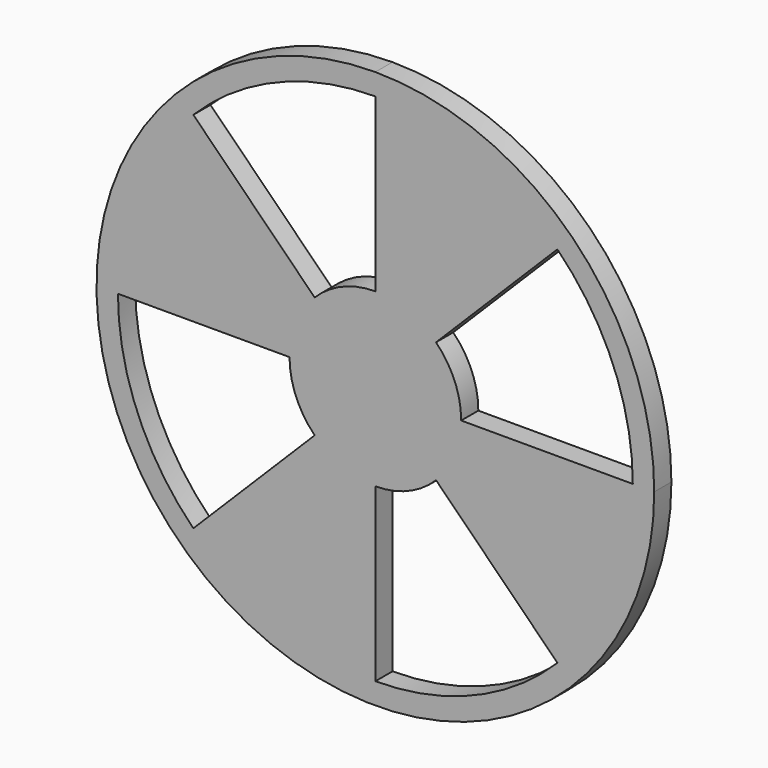
from build123d import *

# Parameters (mm, degrees)
F0_R     = 9.525
F1_DEPTH = 3.175


with BuildPart() as f1:
    # F0 (on Front) → F1 (new body)
    with BuildSketch(Plane.XZ):
        with BuildLine():
            ThreePointArc((41.275, 0), (29.1858323935, 29.1858323935), (0, 41.275))
            ThreePointArc((0, 41.275), (-29.1858323935, -29.1858323935), (41.275, 0))
        make_face()
        with BuildLine():
            ThreePointArc((26.9407683632, 26.9407683632), (35.1998101887, 14.5802387731), (38.1, 0))
            ThreePointArc((38.1, 0), (35.1998101887, -14.5802387731), (26.9407683632, -26.9407683632))
            ThreePointArc((26.9407683632, -26.9407683632), (14.5802387731, -35.1998101887), (0, -38.1))
            ThreePointArc((0, -38.1), (-14.5802387731, -35.1998101887), (-26.9407683632, -26.9407683632))
            ThreePointArc((-26.9407683632, -26.9407683632), (-35.1998101887, -14.5802387731), (-38.1, 0))
            ThreePointArc((-38.1, 0), (-35.1998101887, 14.5802387731), (-26.9407683632, 26.9407683632))
            ThreePointArc((-26.9407683632, 26.9407683632), (-14.5802387731, 35.1998101887), (0, 38.1))
            ThreePointArc((0, 38.1), (14.5802387731, 35.1998101887), (26.9407683632, 26.9407683632))
        make_face(mode=Mode.SUBTRACT)
        with BuildLine():
            ThreePointArc((26.9407683632, -26.9407683632), (35.1998101887, -14.5802387731), (38.1, 0))
            Line((38.1, 0), (12.7, 0))
            ThreePointArc((12.7, 0), (11.7332700629, -4.860079591), (8.9802561211, -8.9802561211))
            Line((8.9802561211, -8.9802561211), (26.9407683632, -26.9407683632))
        make_face()
        with BuildLine():
            Line((8.9802561211, 8.9802561211), (26.9407683632, 26.9407683632))
            ThreePointArc((26.9407683632, 26.9407683632), (14.5802387731, 35.1998101887), (0, 38.1))
            Line((0, 38.1), (0, 12.7))
            ThreePointArc((0, 12.7), (4.860079591, 11.7332700629), (8.9802561211, 8.9802561211))
        make_face()
        with BuildLine():
            ThreePointArc((8.9802561211, -8.9802561211), (11.7332700629, -4.860079591), (12.7, 0))
            ThreePointArc((12.7, 0), (11.7332700629, 4.860079591), (8.9802561211, 8.9802561211))
            ThreePointArc((8.9802561211, 8.9802561211), (4.860079591, 11.7332700629), (0, 12.7))
            ThreePointArc((0, 12.7), (-4.860079591, 11.7332700629), (-8.9802561211, 8.9802561211))
            ThreePointArc((-8.9802561211, 8.9802561211), (-11.7332700629, 4.860079591), (-12.7, 0))
            ThreePointArc((-12.7, 0), (-11.7332700629, -4.860079591), (-8.9802561211, -8.9802561211))
            ThreePointArc((-8.9802561211, -8.9802561211), (-4.860079591, -11.7332700629), (0, -12.7))
            ThreePointArc((0, -12.7), (4.860079591, -11.7332700629), (8.9802561211, -8.9802561211))
        make_face()
        Circle(F0_R, mode=Mode.SUBTRACT)
        with BuildLine():
            ThreePointArc((-26.9407683632, -26.9407683632), (-14.5802387731, -35.1998101887), (0, -38.1))
            Line((0, -38.1), (0, -12.7))
            ThreePointArc((0, -12.7), (-4.860079591, -11.7332700629), (-8.9802561211, -8.9802561211))
            Line((-8.9802561211, -8.9802561211), (-26.9407683632, -26.9407683632))
        make_face()
        with BuildLine():
            Line((-8.9802561211, 8.9802561211), (-26.9407683632, 26.9407683632))
            ThreePointArc((-26.9407683632, 26.9407683632), (-35.1998101887, 14.5802387731), (-38.1, 0))
            Line((-38.1, 0), (-12.7, 0))
            ThreePointArc((-12.7, 0), (-11.7332700629, 4.860079591), (-8.9802561211, 8.9802561211))
        make_face()
        Circle(F0_R)
    extrude(amount=F1_DEPTH)


solid = f1.part
